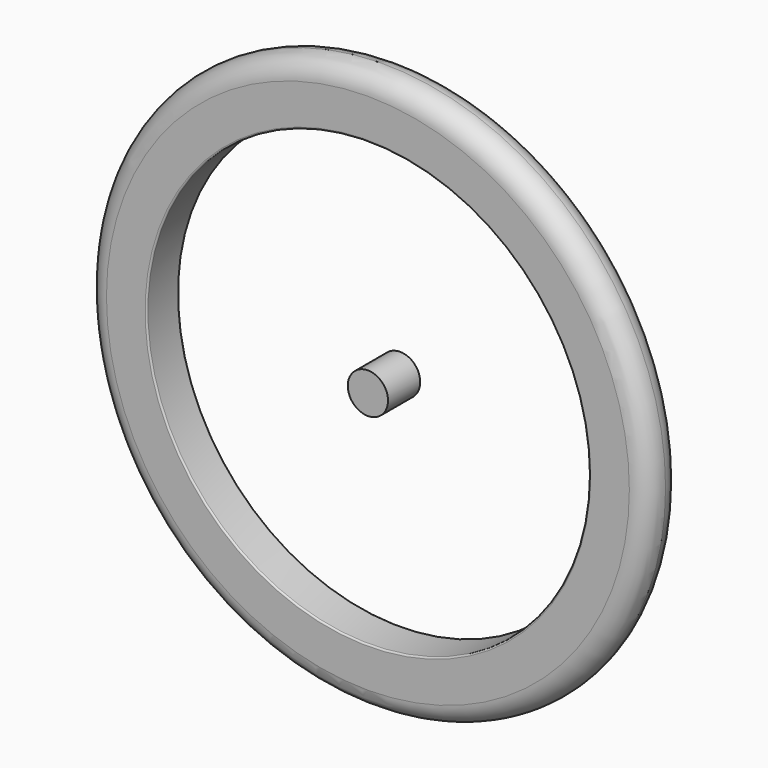
from build123d import *

# Parameters (mm, degrees)
F0_R     = 88.9
F1_DEPTH = 12.7
F2_R     = 69.85
F2_R_2   = 6.35
F3_DEPTH = 25.4
F4_R     = 6.34999
F5_R     = 0.508


# Not quite as in the source:
# - a fillet or chamfer is up to 0.001 mm smaller than in the source, because OpenCascade refuses the exact size


with BuildPart() as f1:
    # F0 (on Front) → F1 (new body)
    with BuildSketch(Plane.XZ):
        Circle(F0_R)
    extrude(amount=F1_DEPTH)

    # F2 (on face) → F3 (cut)
    with BuildSketch(Plane.XZ.offset(12.7)):
        Circle(F2_R)
        Circle(F2_R_2, mode=Mode.SUBTRACT)
    extrude(amount=-F3_DEPTH, mode=Mode.SUBTRACT)

    # F4 (radius 6.35 in the source; OpenCascade refuses exactly that, so slightly less here)
    f4_edges = [f1.edges().sort_by_distance(p)[0] for p in [
        (-88.9, -12.7, 0),
        (-88.9, 0, 0),
    ]]
    fillet(f4_edges, radius=F4_R)

    # F5
    f5_edges = [f1.edges().sort_by_distance(p)[0] for p in [
        (-69.85, 0, 0),
        (-69.85, -12.7, 0),
    ]]
    fillet(f5_edges, radius=F5_R)


solid = f1.part
